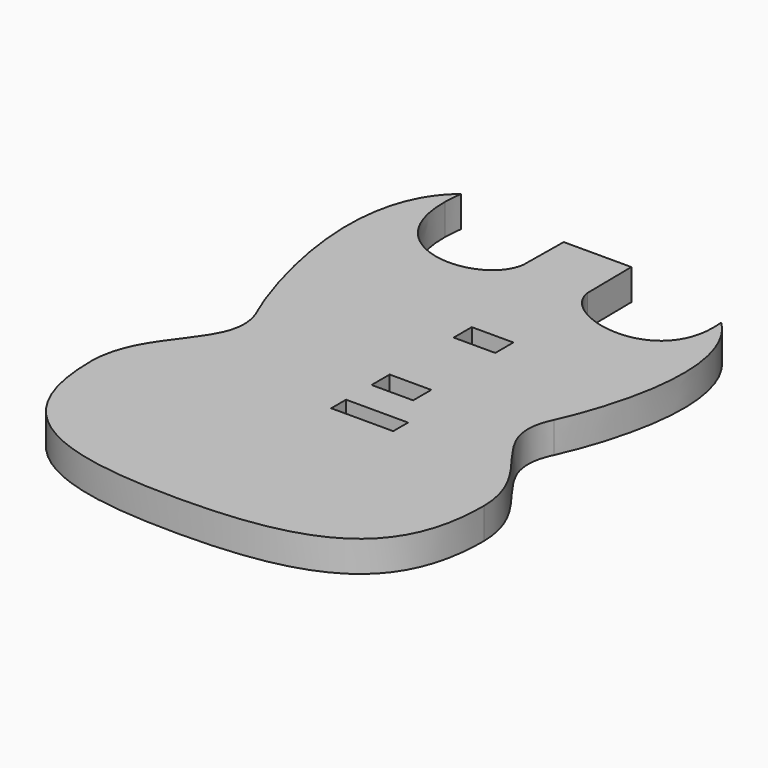
from build123d import *

# Parameters (mm, degrees)
F0_W     = 50
F0_H     = 15
F0_W_2   = 33.55
F0_H_2   = 18.263
F1_DEPTH = 25


# Not quite as in the source:
# - a feature names something its author has since deleted; it is built from what else it names


with BuildPart() as f1:
    # F0 (on Top) → F1 (new body)
    with BuildSketch(Plane.XY):
        Polygon((27.25, 107.8786835152), (-27.25, 107.8786835152), (-27.75, 67.8786835152), (-28.0282922993, 45.6152995713), (-28.25, 27.8786835152), (28.25, 27.8786835152), (28.0907844192, 40.6159299829), (27.8110993763, 62.99073341), align=None)
        with BuildLine():
            Line((-28.0282922993, 45.6152995713), (-27.75, 67.8786835152))
            add(Edge.make_bspline(
                [(-119.8866222784, 104.0838235955), (-121.0423578492, 26.6975843315), (-33.4381163475, 27.9588649836), (-27.75, 67.8786835152)],
                knots=[5.8207414298, 5.8207414298, 5.8207414298, 5.8207414298, 104.177036671, 104.177036671, 104.177036671, 104.177036671], degree=3))
            add(Edge.make_bspline(
                [(-129.4312865498, 88.9177944447), (-128.9681788838, 89.9439533029), (-126.7042715733, 94.6909513961), (-123.5656981618, 99.854792643), (-120.3833088728, 103.5358856243), (-119.8866222778, 104.0838235953)],
                knots=[174.7937382561, 174.7937382561, 174.7937382561, 174.7937382561, 178.1663413599, 190.5368056939, 192.7537167942, 192.7537167942, 192.7537167942, 192.7537167942], degree=3))
            add(Edge.make_bspline(
                [(-129.4312865498, 88.9177944447), (-129.3109849454, 88.0758069), (-128.4336564101, 82.4912333506), (-125.9636072037, 72.6752311218), (-120.2024501307, 60.4880102216), (-112.6215186167, 50.3680139367), (-103.6339611104, 42.3905323107), (-93.696674412, 36.532063254), (-83.2179047221, 32.6896328601), (-72.5392583415, 30.7367375732), (-61.9410573447, 30.5552142432), (-51.6845955009, 32.0994665415), (-42.5038344938, 35.1003258688), (-35.1676094551, 39.272763754), (-30.7048923289, 42.9689824885), (-28.563789449, 45.0637979027), (-28.0282922993, 45.6152995713)],
                knots=[31.2550682463, 31.2550682463, 31.2550682463, 31.2550682463, 33.8015913522, 48.177750167, 61.4744919422, 73.96612477, 85.8554939797, 97.2898755487, 108.3722273852, 119.1669646926, 129.7095146782, 140.0247340346, 150.1520713556, 158.5067230901, 165.1780752822, 167.4830132535, 167.4830132535, 167.4830132535, 167.4830132535], degree=3))
        make_face()
        with BuildLine():
            add(Edge.make_bspline(
                [(27.8110993763, 62.99073341), (32.2933669496, 29.2229355953), (113.1124852102, 12.6623549852), (118.8562015646, 69.1546411271)],
                knots=[0, 0, 0, 0, 86.4138969398, 86.4138969398, 86.4138969398, 86.4138969398], degree=3))
            Line((27.8110993763, 62.99073341), (28.0907844192, 40.6159299829))
            add(Edge.make_bspline(
                [(28.0907844192, 40.6159299829), (29.287798378, 39.3429032121), (32.9148444473, 35.925399713), (39.7570190189, 31.2557479048), (48.6151552623, 26.9252261046), (58.1307163688, 23.8031969869), (68.0898843108, 21.9265931964), (78.3013198669, 21.4068174609), (88.5616997912, 22.40383688), (98.6335430856, 25.1427600429), (108.1809690997, 29.9014168198), (116.6857490885, 36.9285745162), (122.9775786719, 45.5470774874), (125.7269242874, 51.946079615), (126.7237292348, 54.9306006364)],
                knots=[23.8574779363, 23.8574779363, 23.8574779363, 23.8574779363, 29.0928113686, 38.7540016942, 48.5866257781, 58.5851158791, 68.7062096676, 78.9034224293, 89.1584624493, 99.5062924883, 110.045747029, 120.9208868969, 132.2887869108, 141.7007014746, 141.7007014746, 141.7007014746, 141.7007014746], degree=3))
            add(Edge.make_bspline(
                [(126.7237292348, 54.9306006364), (126.1874967207, 56.2317474218), (124.1003720443, 60.9435117835), (121.4166682373, 65.6994419315), (119.0247712369, 68.9308388277), (118.8562015646, 69.1546411271)],
                knots=[140.16898266, 140.16898266, 140.16898266, 140.16898266, 144.3874002602, 155.6048910041, 156.4452003175, 156.4452003175, 156.4452003175, 156.4452003175], degree=3))
        make_face()
        with BuildLine():
            Line((-28.25, 27.8786835152), (-28.0282922993, 45.6152995713))
            add(Edge.make_bspline(
                [(-129.4312865498, 88.9177944447), (-129.3109849454, 88.0758069), (-128.4336564101, 82.4912333506), (-125.9636072037, 72.6752311218), (-120.2024501307, 60.4880102216), (-112.6215186167, 50.3680139367), (-103.6339611104, 42.3905323107), (-93.696674412, 36.532063254), (-83.2179047221, 32.6896328601), (-72.5392583415, 30.7367375732), (-61.9410573447, 30.5552142432), (-51.6845955009, 32.0994665415), (-42.5038344938, 35.1003258688), (-35.1676094551, 39.272763754), (-30.7048923289, 42.9689824885), (-28.563789449, 45.0637979027), (-28.0282922993, 45.6152995713)],
                knots=[31.2550682463, 31.2550682463, 31.2550682463, 31.2550682463, 33.8015913522, 48.177750167, 61.4744919422, 73.96612477, 85.8554939797, 97.2898755487, 108.3722273852, 119.1669646926, 129.7095146782, 140.0247340346, 150.1520713556, 158.5067230901, 165.1780752822, 167.4830132535, 167.4830132535, 167.4830132535, 167.4830132535], degree=3))
            add(Edge.make_bspline(
                [(-130.1583163956, 106.6368603294), (-130.2482463228, 105.1422313843), (-130.4708327377, 99.2283714352), (-130.0575927336, 93.3012938045), (-129.4312865498, 88.9177944447)],
                knots=[13.5070543021, 13.5070543021, 13.5070543021, 13.5070543021, 17.9975296122, 31.2550682463, 31.2550682463, 31.2550682463, 31.2550682463], degree=3))
            add(Edge.make_bspline(
                [(-119.5249942189, -85.1707845054), (-126.9605969931, -69.461302998), (-172.4103162726, 49.7161929114), (-130.1583163912, 106.6368603279)],
                knots=[0, 0, 0, 0, 189.1875471614, 189.1875471614, 189.1875471614, 189.1875471614], degree=3))
            add(Edge.make_bspline(
                [(-158.25, -204.448345688), (-157.6418556412, -147.7076234473), (-96.9115691033, -132.1890450103), (-119.5249942189, -85.1707845054)],
                knots=[0, 0, 0, 0, 125.406390086, 125.406390086, 125.406390086, 125.406390086], degree=3))
            add(Edge.make_bspline(
                [(-158.25, -204.448345688), (-158.25, -290.2131974697), (-106.7391799071, -316.9097596875), (0, -316.9097596875)],
                knots=[0, 0, 0, 0, 194.1407534207, 194.1407534207, 194.1407534207, 194.1407534207], degree=3))
            add(Edge.make_bspline(
                [(158.25, -204.448345688), (158.25, -290.2131974697), (106.7391799071, -316.9097596875), (0, -316.9097596875)],
                knots=[0, 0, 0, 0, 194.1407534207, 194.1407534207, 194.1407534207, 194.1407534207], degree=3))
            add(Edge.make_bspline(
                [(158.25, -204.448345688), (157.6418556412, -147.7076234473), (96.9115691033, -132.1890450103), (119.5249942189, -85.1707845054)],
                knots=[0, 0, 0, 0, 125.406390086, 125.406390086, 125.406390086, 125.406390086], degree=3))
            add(Edge.make_bspline(
                [(119.5249942189, -85.1707845054), (126.5438310067, -70.3415708106), (163.0129687478, 16.9513401574), (129.6580469223, 70.4506637657)],
                knots=[0, 0, 0, 0, 155.1840675903, 155.1840675903, 155.1840675903, 155.1840675903], degree=3))
            add(Edge.make_bspline(
                [(126.7237292348, 54.9306006364), (127.0043283083, 55.7707387556), (128.5538224017, 60.8007183147), (129.4403792123, 66.0439240135), (129.6568620638, 70.4263535727), (129.6580469223, 70.4506637657)],
                knots=[141.7007014746, 141.7007014746, 141.7007014746, 141.7007014746, 144.3501410806, 157.4352190661, 157.5082077989, 157.5082077989, 157.5082077989, 157.5082077989], degree=3))
            add(Edge.make_bspline(
                [(28.0907844192, 40.6159299829), (29.287798378, 39.3429032121), (32.9148444473, 35.925399713), (39.7570190189, 31.2557479048), (48.6151552623, 26.9252261046), (58.1307163688, 23.8031969869), (68.0898843108, 21.9265931964), (78.3013198669, 21.4068174609), (88.5616997912, 22.40383688), (98.6335430856, 25.1427600429), (108.1809690997, 29.9014168198), (116.6857490885, 36.9285745162), (122.9775786719, 45.5470774874), (125.7269242874, 51.946079615), (126.7237292348, 54.9306006364)],
                knots=[23.8574779363, 23.8574779363, 23.8574779363, 23.8574779363, 29.0928113686, 38.7540016942, 48.5866257781, 58.5851158791, 68.7062096676, 78.9034224293, 89.1584624493, 99.5062924883, 110.045747029, 120.9208868969, 132.2887869108, 141.7007014746, 141.7007014746, 141.7007014746, 141.7007014746], degree=3))
            Line((28.0907844192, 40.6159299829), (28.25, 27.8786835152))
            Line((28.25, 27.8786835152), (-28.25, 27.8786835152))
        make_face()
        with Locations((25, -153.0963164848)):
            Rectangle(F0_W, F0_H, mode=Mode.SUBTRACT)
        Polygon((0, -119.9348074679), (0, -101.6718074679), (27.3104757071, -101.6718074679), (33.55, -101.6718074679), (33.55, -119.9348074679), align=None, mode=Mode.SUBTRACT)
        with Locations((16.775, -28.0059413371)):
            Rectangle(F0_W_2, F0_H_2, mode=Mode.SUBTRACT)
        with BuildLine():
            add(Edge.make_bspline(
                [(-129.4312865498, 88.9177944447), (-128.9681788838, 89.9439533029), (-126.7042715733, 94.6909513961), (-123.5656981618, 99.854792643), (-120.3833088728, 103.5358856243), (-119.8866222778, 104.0838235953)],
                knots=[174.7937382561, 174.7937382561, 174.7937382561, 174.7937382561, 178.1663413599, 190.5368056939, 192.7537167942, 192.7537167942, 192.7537167942, 192.7537167942], degree=3))
            add(Edge.make_bspline(
                [(-118.7134671008, 118.6576419779), (-119.4389657293, 113.5187304004), (-119.8182256607, 108.6635537275), (-119.8866222784, 104.0838235955)],
                knots=[0, 0, 0, 0, 5.8207414298, 5.8207414298, 5.8207414298, 5.8207414298], degree=3))
            add(Edge.make_bspline(
                [(-130.1583163912, 106.6368603279), (-126.888150362, 111.0423330505), (-123.0926289669, 115.0748717049), (-118.7134671008, 118.6576419779)],
                knots=[189.1875471614, 189.1875471614, 189.1875471614, 189.1875471614, 203.8300419931, 203.8300419931, 203.8300419931, 203.8300419931], degree=3))
            add(Edge.make_bspline(
                [(-130.1583163956, 106.6368603294), (-130.2482463228, 105.1422313843), (-130.4708327377, 99.2283714352), (-130.0575927336, 93.3012938045), (-129.4312865498, 88.9177944447)],
                knots=[13.5070543021, 13.5070543021, 13.5070543021, 13.5070543021, 17.9975296122, 31.2550682463, 31.2550682463, 31.2550682463, 31.2550682463], degree=3))
        make_face()
        with BuildLine():
            add(Edge.make_bspline(
                [(118.8562015646, 69.1546411271), (119.3162948222, 73.679885474), (119.2946583668, 78.6738817109), (118.7134671008, 84.1653342065)],
                knots=[86.4138969398, 86.4138969398, 86.4138969398, 86.4138969398, 93.3359747193, 93.3359747193, 93.3359747193, 93.3359747193], degree=3))
            add(Edge.make_bspline(
                [(126.7237292348, 54.9306006364), (126.1874967207, 56.2317474218), (124.1003720443, 60.9435117835), (121.4166682373, 65.6994419315), (119.0247712369, 68.9308388277), (118.8562015646, 69.1546411271)],
                knots=[140.16898266, 140.16898266, 140.16898266, 140.16898266, 144.3874002602, 155.6048910041, 156.4452003175, 156.4452003175, 156.4452003175, 156.4452003175], degree=3))
            add(Edge.make_bspline(
                [(126.7237292348, 54.9306006364), (127.0043283083, 55.7707387556), (128.5538224017, 60.8007183147), (129.4403792123, 66.0439240135), (129.6568620638, 70.4263535727), (129.6580469223, 70.4506637657)],
                knots=[141.7007014746, 141.7007014746, 141.7007014746, 141.7007014746, 144.3501410806, 157.4352190661, 157.5082077989, 157.5082077989, 157.5082077989, 157.5082077989], degree=3))
            add(Edge.make_bspline(
                [(129.6580469223, 70.4506637657), (126.6158182503, 75.3302187852), (122.992732948, 79.9286496563), (118.7134671008, 84.1653342065)],
                knots=[155.1840675903, 155.1840675903, 155.1840675903, 155.1840675903, 169.3380632837, 169.3380632837, 169.3380632837, 169.3380632837], degree=3))
        make_face()
    extrude(amount=F1_DEPTH)


solid = f1.part
